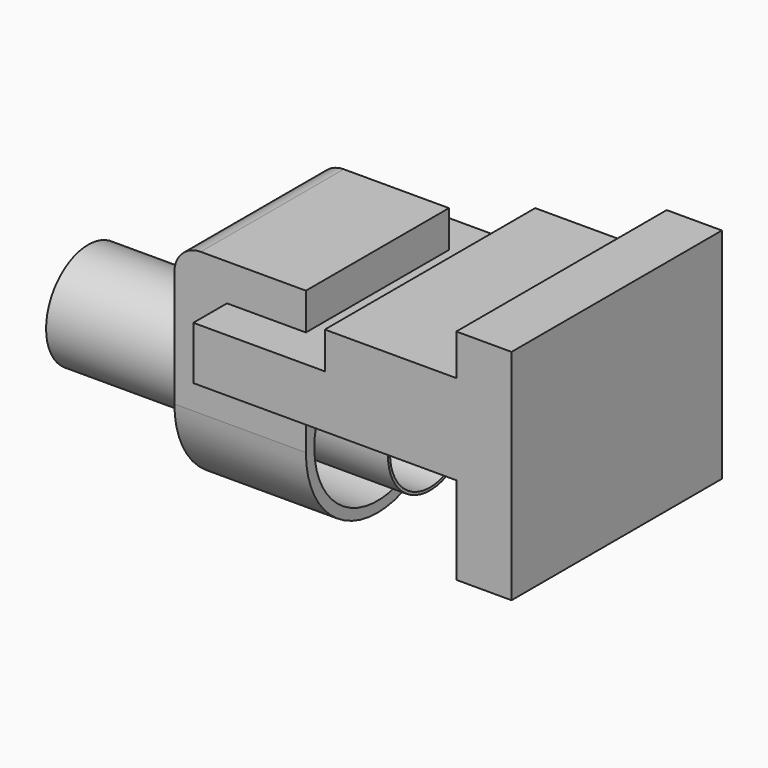
from build123d import *

# Parameters (mm, degrees)
F0_W          = 25
F0_H          = 7
F0_W_2        = 10.5
F0_H_2        = 16.6735936701
F0_H_3        = 10.1
F0_H_4        = 7.8
F1_DEPTH      = 25
F1_DEPTH_BACK = 25
F2_R          = 10
F2_R_2        = 9.5
F3_DEPTH      = 40
F3_DEPTH_BACK = 25
F4_W          = 34
F4_H          = 7
F5_DEPTH      = 10
F6_W          = 34
F6_H          = 7
F7_DEPTH      = 15
F8_R          = 5


with BuildPart() as f1:
    # F0 (on Front) → F1 (new body, two sides)
    with BuildSketch(Plane.XZ) as f1_sk:
        with Locations((7, 8.6)):
            Rectangle(F0_W, F0_H)
        with Locations((24.75, -13.3367968351)):
            Rectangle(F0_W_2, F0_H_2)
        with Locations((24.75, 0.05)):
            Rectangle(F0_W_2, F0_H_3)
        with Locations((24.75, 16)):
            Rectangle(F0_W_2, F0_H_4)
        with Locations((24.75, 8.6)):
            Rectangle(F0_W_2, F0_H)
        Polygon((-5.5, 5.1), (-30.5, 5.1), (-30.5, -5), (19.5, -5), (19.5, 5.1), align=None)
    extrude(amount=F1_DEPTH)
    extrude(f1_sk.sketch, amount=-F1_DEPTH_BACK)


with BuildPart() as f3:
    # F2 (on face) → F3 (new body, two sides)
    with BuildSketch(Plane(origin=(-30.5, 0, 0), x_dir=(0, -1, 0), z_dir=(-1, 0, 0))) as f3_sk:
        with Locations((0, -15)):
            Circle(F2_R)
        with Locations((0, -15)):
            Circle(F2_R_2, mode=Mode.SUBTRACT)
    extrude(amount=F3_DEPTH)
    extrude(f3_sk.sketch, amount=-F3_DEPTH_BACK)


with BuildPart() as f5:
    # F4 (on face) → F5 (new body)
    with BuildSketch(Plane(origin=(-30.5, 0, 0), x_dir=(0, -1, 0), z_dir=(-1, 0, 0))):
        with BuildLine():
            ThreePointArc((11.1803398875, -5), (14.0125853844, -9.6476686534), (15, -15))
            ThreePointArc((15, -15), (-5.3523313466, -29.0125853844), (-11.1803398875, -5))
            Line((-11.1803398875, -5), (-13.7477270849, -5))
            ThreePointArc((-13.7477270849, -5), (-16.1664987001, -9.7422134145), (-17, -15))
            ThreePointArc((-17, -15), (0, -32), (17, -15))
            ThreePointArc((17, -15), (16.1664987001, -9.7422134145), (13.7477270849, -5))
            Line((13.7477270849, -5), (11.1803398875, -5))
        make_face()
        with BuildLine():
            ThreePointArc((-17, -15), (-16.1664987001, -9.7422134145), (-13.7477270849, -5))
            Line((-13.7477270849, -5), (-17, -5))
            Line((-17, -5), (-17, -15))
        make_face()
        with BuildLine():
            Line((17, -5), (13.7477270849, -5))
            ThreePointArc((13.7477270849, -5), (16.1664987001, -9.7422134145), (17, -15))
            Line((17, -15), (17, -5))
        make_face()
        with BuildLine():
            ThreePointArc((-13.7477270849, -5), (0, 2), (13.7477270849, -5))
            Line((13.7477270849, -5), (17, -5))
            Line((17, -5), (17, 5.1))
            Line((17, 5.1), (-17, 5.1))
            Line((-17, 5.1), (-17, -5))
            Line((-17, -5), (-13.7477270849, -5))
        make_face()
        with BuildLine():
            ThreePointArc((-11.1803398875, -5), (0, 0), (11.1803398875, -5))
            Line((11.1803398875, -5), (13.7477270849, -5))
            ThreePointArc((13.7477270849, -5), (0, 2), (-13.7477270849, -5))
            Line((-13.7477270849, -5), (-11.1803398875, -5))
        make_face()
        with BuildLine():
            Line((-11.1803398875, -5), (11.1803398875, -5))
            ThreePointArc((11.1803398875, -5), (0, 0), (-11.1803398875, -5))
        make_face()
        with Locations((0, 8.6)):
            Rectangle(F4_W, F4_H)
    extrude(amount=F5_DEPTH)

    # F6 (on face) → F7 (join)
    with BuildSketch(Plane.YZ.offset(-30.5)):
        with Locations((0, 8.6)):
            Rectangle(F6_W, F6_H)
        with BuildLine():
            Line((17, -15), (17, -5))
            Line((17, -5), (11.1803398875, -5))
            ThreePointArc((11.1803398875, -5), (0, -30), (-11.1803398875, -5))
            Line((-11.1803398875, -5), (-17, -5))
            Line((-17, -5), (-17, -15))
            ThreePointArc((-17, -15), (0, -32), (17, -15))
        make_face()
    extrude(amount=F7_DEPTH)

    # F8
    f8_edges = [f5.edges().sort_by_distance(p)[0] for p in [
        (-40.5, 0, 12.1),
    ]]
    fillet(f8_edges, radius=F8_R)


solid = Compound([f1.part, f3.part, f5.part])
